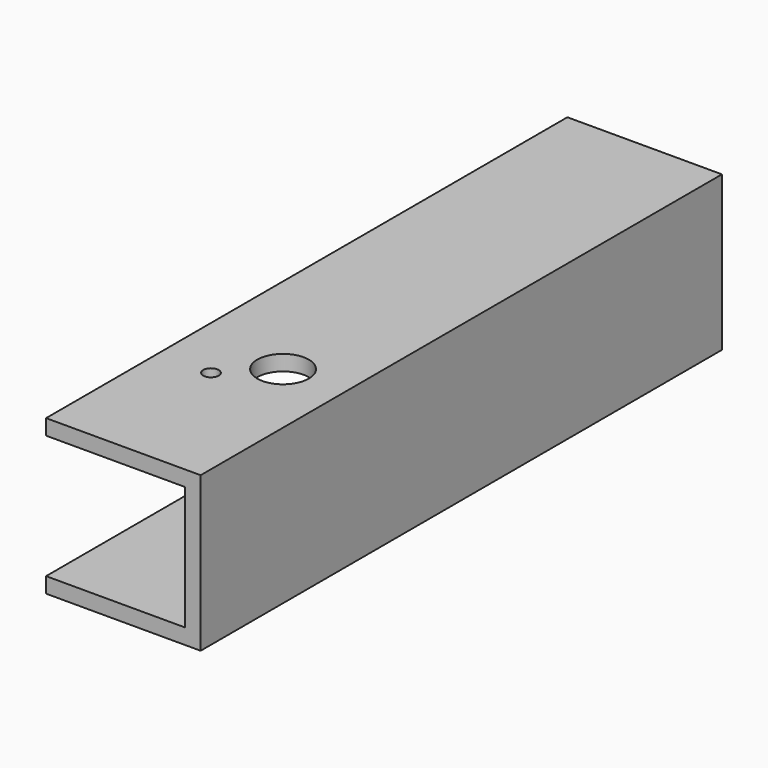
from build123d import *

# Parameters (mm, degrees)
F0_W     = 30
F0_H     = 126.4803184569
F1_DEPTH = 3
F2_W     = 3
F2_H     = 126.4803184569
F3_DEPTH = 30
F4_START = -24
F4_DEPTH = 3


with BuildPart() as f1:
    # F0 (on Top) → F1 (new body)
    with BuildSketch(Plane.XY):
        with Locations((-3, 28.2401592284)):
            Rectangle(F0_W, F0_H)
        with BuildLine():
            ThreePointArc((-6.2781745931, -7.7781745931), (-9.1639938918, -8.3521997416), (-6.7175144213, -6.7175144213))
            ThreePointArc((-6.7175144213, -6.7175144213), (-6.3923552943, -7.2041494445), (-6.2781745931, -7.7781745931))
        make_face(mode=Mode.SUBTRACT)
        with BuildLine():
            ThreePointArc((-3.5355339059, -3.5355339059), (-1.9134171618, 4.6193976626), (5, 0))
            ThreePointArc((5, 0), (1.9134171618, -4.6193976626), (-3.5355339059, -3.5355339059))
        make_face(mode=Mode.SUBTRACT)
    extrude(amount=F1_DEPTH)

    # F2 (on face) → F3 (join)
    with BuildSketch(Plane.XY.offset(3)):
        with Locations((10.5, 28.2401592284)):
            Rectangle(F2_W, F2_H)
    extrude(amount=-F3_DEPTH)

    # F0 (on Top) → F4 (join)
    with BuildSketch(Plane.XY.offset(F4_START)):
        with Locations((-3, 28.2401592284)):
            Rectangle(F0_W, F0_H)
        with BuildLine():
            ThreePointArc((-6.2781745931, -7.7781745931), (-9.1639938918, -8.3521997416), (-6.7175144213, -6.7175144213))
            ThreePointArc((-6.7175144213, -6.7175144213), (-6.3923552943, -7.2041494445), (-6.2781745931, -7.7781745931))
        make_face(mode=Mode.SUBTRACT)
        with BuildLine():
            ThreePointArc((-3.5355339059, -3.5355339059), (-1.9134171618, 4.6193976626), (5, 0))
            ThreePointArc((5, 0), (1.9134171618, -4.6193976626), (-3.5355339059, -3.5355339059))
        make_face(mode=Mode.SUBTRACT)
        with BuildLine():
            ThreePointArc((-3.5355339059, -3.5355339059), (1.9134171618, -4.6193976626), (5, 0))
            ThreePointArc((5, 0), (-1.9134171618, 4.6193976626), (-3.5355339059, -3.5355339059))
        make_face()
        with BuildLine():
            ThreePointArc((-6.2781745931, -7.7781745931), (-6.3923552943, -7.2041494445), (-6.7175144213, -6.7175144213))
            ThreePointArc((-6.7175144213, -6.7175144213), (-9.1639938918, -8.3521997416), (-6.2781745931, -7.7781745931))
        make_face()
    extrude(amount=-F4_DEPTH)


solid = f1.part
